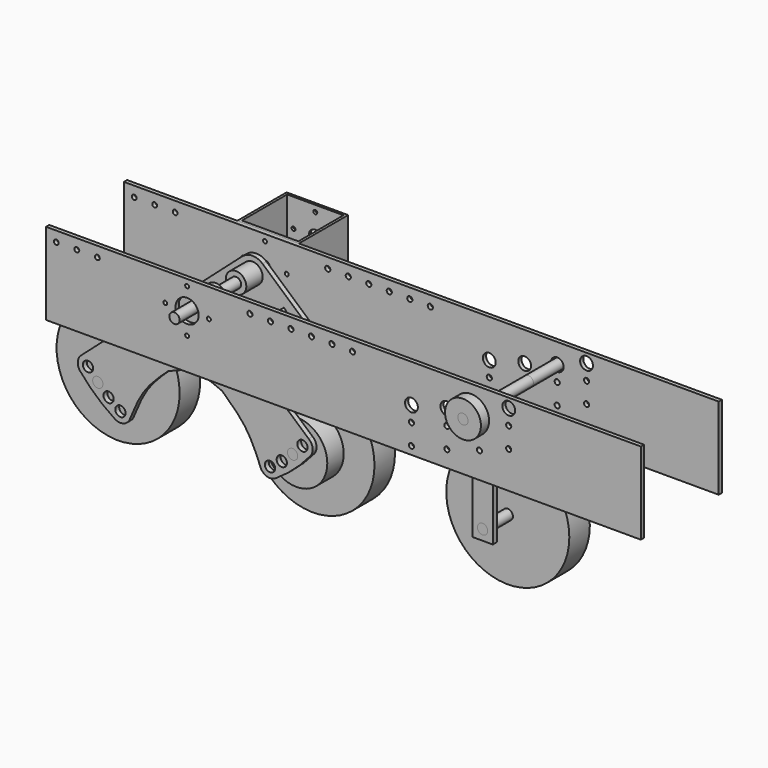
from build123d import *

# Parameters (mm, degrees)
F1_R           = 76.2
F1_R_2         = 6.35
F2_DEPTH       = 31.75
F3_R           = 38.1
F3_R_2         = 6.35
F4_DEPTH       = 25.4
F5_R           = 38.1
F5_R_2         = 6.35
F6_DEPTH       = 25.4
F0_R           = 6.35
F7_DEPTH       = 25.4
F7_DEPTH_BACK  = 57.15
F8_R           = 12.7
F8_R_2         = 6.35
F9_DEPTH       = 25.4
F10_R          = 12.7
F10_R_2        = 6.35
F11_DEPTH      = 25.4
F12_R          = 6.35
F13_DEPTH      = 6.0452
F14_R          = 6.35
F14_R_2        = 3.175
F15_DEPTH      = 6.0452
F18_W          = 736.6
F18_H          = 101.6
F18_R          = 2.4257
F18_R_2        = 3.175
F18_R_3        = 6.35
F18_R_4        = 2.983685919
F18_R_5        = 7.9375
F19_DEPTH      = 4.9403
F21_W          = 736.6
F21_H          = 101.6
F21_R          = 2.4257
F21_R_2        = 3.175
F21_R_3        = 14.2875
F21_R_4        = 2.983685919
F21_R_5        = 7.9375
F22_DEPTH      = 4.9403
F23_R          = 22.225
F24_DEPTH      = 11.43
F26_W          = 25.4
F26_H          = 6.35
F27_DEPTH      = 12.7
F27_DEPTH_BACK = 152.4
F28_R          = 6.35
F28_R_2        = 7.9375
F28_R_3        = 3.175
F29_DEPTH      = 126.8603
F30_W          = 76.2
F30_H          = 76.2
F30_W_2        = 69.85
F30_H_2        = 69.85
F31_DEPTH      = 69.85
F32_R          = 2.4257
F32_R_2        = 7.9375
F33_DEPTH      = 76.2
F34_R          = 6.35
F35_DEPTH      = 56.0451
F35_DEPTH_BACK = 75.7555
F36_DEPTH      = 25.4
F37_R          = 22.225
F37_R_2        = 6.35
F38_DEPTH      = 12.7
F39_DEPTH      = 38.1
F40_R          = 6.35
F41_DEPTH      = 126.8603
F42_R          = 6.35
F43_DEPTH      = 94.6404
F44_DEPTH      = 50.8
F45_R          = 3.175
F46_DEPTH      = 82.55


with BuildPart() as f2:
    # F1 (on Front) → F2 (new body)
    with BuildSketch(Plane.XZ):
        Circle(F1_R)
        Circle(F1_R_2, mode=Mode.SUBTRACT)
    extrude(amount=F2_DEPTH)


with BuildPart() as f2b:
    # F1 (on Front) → F2, piece 2 (new body)
    with BuildSketch(Plane.XZ):
        with Locations((241.3, 0)):
            Circle(F1_R)
        with Locations((241.3, 0)):
            Circle(F1_R_2, mode=Mode.SUBTRACT)
    extrude(amount=F2_DEPTH)


with BuildPart() as f2c:
    # F1 (on Front) → F2, piece 3 (new body)
    with BuildSketch(Plane.XZ):
        with Locations((482.6, 0.0227596388)):
            Circle(F1_R)
        with Locations((482.6, 0.0227596388)):
            Circle(F1_R_2, mode=Mode.SUBTRACT)
    extrude(amount=F2_DEPTH)


with BuildPart() as f4:
    # F3 (on face) → F4 (new body)
    with BuildSketch(Plane.XZ):
        Circle(F3_R)
        Circle(F3_R_2, mode=Mode.SUBTRACT)
    extrude(amount=-F4_DEPTH)


with BuildPart() as f6:
    # F5 (on face) → F6 (new body)
    with BuildSketch(Plane.XZ.offset(31.75)):
        with Locations((241.3, 0)):
            Circle(F5_R)
        with Locations((241.3, 0)):
            Circle(F5_R_2, mode=Mode.SUBTRACT)
    extrude(amount=F6_DEPTH)


with BuildPart() as f7:
    # F0 (on Front) → F7 (new body, two sides)
    with BuildSketch(Plane.XZ) as f7_sk:
        with Locations((120.65, 122.1713596388)):
            Circle(F0_R)
    extrude(amount=-F7_DEPTH)
    extrude(f7_sk.sketch, amount=F7_DEPTH_BACK)

    # F39 (add): a face of the model
    f39_faces = [f7.faces().sort_by_distance(p)[0] for p in [
        (120.65, -57.15, 122.1713596388),
    ]]
    extrude(f39_faces, amount=F39_DEPTH)


with BuildPart() as f9:
    # F8 (on face) → F9 (new body)
    with BuildSketch(Plane.XZ.offset(57.15)):
        with Locations((120.65, 122.1713596388)):
            Circle(F8_R)
        with Locations((120.65, 122.1713596388)):
            Circle(F8_R_2, mode=Mode.SUBTRACT)
    extrude(amount=-F9_DEPTH)


with BuildPart() as f11:
    # F10 (on face) → F11 (new body)
    with BuildSketch(Plane(origin=(0, 25.4, 0), x_dir=(-1, 0, 0), z_dir=(0, 1, 0))):
        with Locations((-120.65, 122.1713596388)):
            Circle(F10_R)
        with Locations((-120.65, 122.1713596388)):
            Circle(F10_R_2, mode=Mode.SUBTRACT)
    extrude(amount=-F11_DEPTH)


with BuildPart() as f13:
    # F12 (on face) → F13 (new body)
    with BuildSketch(Plane(origin=(0, 25.4, 0), x_dir=(-1, 0, 0), z_dir=(0, 1, 0))):
        with BuildLine():
            Line((-133.2704333117, 136.4411586221), (-261.0948431927, 23.3912521446))
            ThreePointArc((-261.0948431927, 23.3912521446), (-266.0226994754, 14.7625060658), (-263.2289371867, 5.2265782815))
            ThreePointArc((-263.2289371867, 5.2265782815), (-243.1793595629, -15.6378971661), (-220.112702455, -33.1090513484))
            ThreePointArc((-220.112702455, -33.1090513484), (-210.3154284268, -34.7681016947), (-202.3223963934, -28.864673424))
            add(Edge.make_bspline(
                [(-202.3223963934, -28.864673424), (-196.8876219657, -15.4698153256), (-186.0180731103, 11.3199008713), (-164.7164012291, 30.8666336238), (-154.0655652885, 40.64)],
                knots=[0, 0, 0, 0, 0.5, 1, 1, 1, 1], degree=3))
            add(Edge.make_bspline(
                [(-154.0655652885, 40.64), (-142.9270435257, 45.4025), (-120.65, 54.9275), (-98.3729564743, 45.4025), (-87.2344347115, 40.64)],
                knots=[0, 0, 0, 0, 0.5, 1, 1, 1, 1], degree=3))
            add(Edge.make_bspline(
                [(-87.2344347115, 40.64), (-76.5835987709, 30.8666336238), (-55.2819268897, 11.3199008713), (-44.4123780343, -15.4698153256), (-38.9776036066, -28.864673424)],
                knots=[0, 0, 0, 0, 0.5, 1, 1, 1, 1], degree=3))
            ThreePointArc((-38.9776036066, -28.864673424), (-30.9845715732, -34.7681016947), (-21.187297545, -33.1090513484))
            ThreePointArc((-21.187297545, -33.1090513484), (1.8793595629, -15.6378971661), (21.9289371867, 5.2265782815))
            ThreePointArc((21.9289371867, 5.2265782815), (24.7226994754, 14.7625060658), (19.7948431927, 23.3912521446))
            Line((19.7948431927, 23.3912521446), (-108.0295666883, 136.4411586221))
            ThreePointArc((-108.0295666883, 136.4411586221), (-120.65, 141.2213596388), (-133.2704333117, 136.4411586221))
        make_face()
        with Locations((-213.2626540765, -22.4148081674)):
            Circle(F12_R, mode=Mode.SUBTRACT)
        with Locations((-241.3, 0)):
            Circle(F12_R, mode=Mode.SUBTRACT)
        with Locations((-227.8686821978, -11.9420916021)):
            Circle(F12_R, mode=Mode.SUBTRACT)
        with Locations((-253.4094511545, 13.2806265843)):
            Circle(F12_R, mode=Mode.SUBTRACT)
        with Locations((-28.0373459235, -22.4148081674)):
            Circle(F12_R, mode=Mode.SUBTRACT)
        with Locations((-13.4313178022, -11.9420916021)):
            Circle(F12_R, mode=Mode.SUBTRACT)
        Circle(F12_R, mode=Mode.SUBTRACT)
        with Locations((12.1094511545, 13.2806265843)):
            Circle(F12_R, mode=Mode.SUBTRACT)
        with Locations((-120.65, 122.1713596388)):
            Circle(F12_R, mode=Mode.SUBTRACT)
    extrude(amount=F13_DEPTH)


with BuildPart() as f15:
    # F14 (on face) → F15 (new body)
    with BuildSketch(Plane.XZ.offset(57.15)):
        with BuildLine():
            ThreePointArc((133.2704333117, 136.4411586221), (120.65, 141.2213596388), (108.0295666883, 136.4411586221))
            Line((108.0295666883, 136.4411586221), (-19.7948431927, 23.3912521446))
            ThreePointArc((-19.7948431927, 23.3912521446), (-24.7226994754, 14.7625060658), (-21.9289371867, 5.2265782815))
            ThreePointArc((-21.9289371867, 5.2265782815), (-1.8793595629, -15.6378971661), (21.187297545, -33.1090513484))
            ThreePointArc((21.187297545, -33.1090513484), (30.9845715732, -34.7681016947), (38.9776036066, -28.864673424))
            add(Edge.make_bspline(
                [(38.9776036066, -28.864673424), (44.4123780343, -15.4698153256), (55.2819268897, 11.3199008713), (76.5835987709, 30.8666336238), (87.2344347115, 40.64)],
                knots=[0, 0, 0, 0, 0.5, 1, 1, 1, 1], degree=3))
            add(Edge.make_bspline(
                [(87.2344347115, 40.64), (98.3729564743, 45.4025), (120.65, 54.9275), (142.9270435257, 45.4025), (154.0655652885, 40.64)],
                knots=[0, 0, 0, 0, 0.5, 1, 1, 1, 1], degree=3))
            add(Edge.make_bspline(
                [(154.0655652885, 40.64), (164.7164012291, 30.8666336238), (186.0180731103, 11.3199008713), (196.8876219657, -15.4698153256), (202.3223963934, -28.864673424)],
                knots=[0, 0, 0, 0, 0.5, 1, 1, 1, 1], degree=3))
            ThreePointArc((202.3223963934, -28.864673424), (210.3154284268, -34.7681016947), (220.112702455, -33.1090513484))
            ThreePointArc((220.112702455, -33.1090513484), (243.1793595629, -15.6378971661), (263.2289371867, 5.2265782815))
            ThreePointArc((263.2289371867, 5.2265782815), (266.0226994754, 14.7625060658), (261.0948431927, 23.3912521446))
            Line((261.0948431927, 23.3912521446), (133.2704333117, 136.4411586221))
        make_face()
        with Locations((28.0373459235, -22.4148081674)):
            Circle(F14_R, mode=Mode.SUBTRACT)
        Circle(F14_R, mode=Mode.SUBTRACT)
        with Locations((13.4313178022, -11.9420916021)):
            Circle(F14_R, mode=Mode.SUBTRACT)
        with Locations((-12.1094511545, 13.2806265843)):
            Circle(F14_R, mode=Mode.SUBTRACT)
        with Locations((213.2626540765, -22.4148081674)):
            Circle(F14_R, mode=Mode.SUBTRACT)
        with Locations((227.8686821978, -11.9420916021)):
            Circle(F14_R, mode=Mode.SUBTRACT)
        with Locations((241.3, 0)):
            Circle(F14_R, mode=Mode.SUBTRACT)
        with Locations((253.4094511545, 13.2806265843)):
            Circle(F14_R, mode=Mode.SUBTRACT)
        with Locations((65.7991565264, 60.479484402)):
            Circle(F14_R_2, mode=Mode.SUBTRACT)
        with Locations((82.6763391337, 79.4615998595)):
            Circle(F14_R_2, mode=Mode.SUBTRACT)
        with Locations((99.5535217409, 98.443715317)):
            Circle(F14_R_2, mode=Mode.SUBTRACT)
        with Locations((120.65, 122.1713596388)):
            Circle(F14_R, mode=Mode.SUBTRACT)
        with Locations((175.5008434736, 60.479484402)):
            Circle(F14_R_2, mode=Mode.SUBTRACT)
        with Locations((158.6236608663, 79.4615998595)):
            Circle(F14_R_2, mode=Mode.SUBTRACT)
        with Locations((141.7464782591, 98.443715317)):
            Circle(F14_R_2, mode=Mode.SUBTRACT)
    extrude(amount=F15_DEPTH)


with BuildPart() as f19:
    # F18 (on offset) → F19 (new body)
    with BuildSketch(Plane.XZ.offset(-44.7548)):
        with Locations((314.325, 106.2963596388)):
            Rectangle(F18_W, F18_H)
        with Locations((120.65, 95.1838596388)):
            Circle(F18_R, mode=Mode.SUBTRACT)
        with Locations((398.4861859235, 65.4437918326)):
            Circle(F18_R_2, mode=Mode.SUBTRACT)
        with Locations((442.3052378022, 75.9165083979)):
            Circle(F18_R_2, mode=Mode.SUBTRACT)
        with Locations((398.4861859235, 90.8437918326)):
            Circle(F18_R_2, mode=Mode.SUBTRACT)
        with Locations((482.6, 87.8586)):
            Circle(F18_R_2, mode=Mode.SUBTRACT)
        with Locations((442.3052378022, 101.3165083979)):
            Circle(F18_R_2, mode=Mode.SUBTRACT)
        with Locations((518.9283488455, 101.1392265843)):
            Circle(F18_R_2, mode=Mode.SUBTRACT)
        with Locations((93.6625, 122.1713596388)):
            Circle(F18_R, mode=Mode.SUBTRACT)
        with Locations((120.65, 122.1713596388)):
            Circle(F18_R_3, mode=Mode.SUBTRACT)
        with Locations((147.6375, 122.1713596388)):
            Circle(F18_R, mode=Mode.SUBTRACT)
        with Locations((-41.275, 144.3963596388)):
            Circle(F18_R_4, mode=Mode.SUBTRACT)
        with Locations((-15.875, 144.3963596388)):
            Circle(F18_R_4, mode=Mode.SUBTRACT)
        with Locations((9.525, 144.3963596388)):
            Circle(F18_R_4, mode=Mode.SUBTRACT)
        with Locations((120.65, 149.1588596388)):
            Circle(F18_R, mode=Mode.SUBTRACT)
        with Locations((198.4375, 144.3963596388)):
            Circle(F18_R_2, mode=Mode.SUBTRACT)
        with Locations((223.8375, 144.3963596388)):
            Circle(F18_R_2, mode=Mode.SUBTRACT)
        with Locations((249.2375, 144.3963596388)):
            Circle(F18_R_2, mode=Mode.SUBTRACT)
        with Locations((274.6375, 144.3963596388)):
            Circle(F18_R_2, mode=Mode.SUBTRACT)
        with Locations((300.0375, 144.3963596388)):
            Circle(F18_R_2, mode=Mode.SUBTRACT)
        with Locations((398.4861859235, 109.8937918326)):
            Circle(F18_R_5, mode=Mode.SUBTRACT)
        with Locations((482.6, 113.2586)):
            Circle(F18_R_2, mode=Mode.SUBTRACT)
        with Locations((442.3052378022, 120.3665083979)):
            Circle(F18_R_5, mode=Mode.SUBTRACT)
        with Locations((518.9283488455, 126.5392265843)):
            Circle(F18_R_2, mode=Mode.SUBTRACT)
        with Locations((482.6, 132.3086)):
            Circle(F18_R_5, mode=Mode.SUBTRACT)
        with Locations((325.4375, 144.3963596388)):
            Circle(F18_R_2, mode=Mode.SUBTRACT)
        with Locations((518.9283488455, 145.5892265843)):
            Circle(F18_R_5, mode=Mode.SUBTRACT)
    extrude(amount=-F19_DEPTH)


with BuildPart() as f22:
    # F21 (on offset) → F22 (new body)
    with BuildSketch(Plane.XZ.offset(70.8152)):
        with Locations((314.325, 106.2963596388)):
            Rectangle(F21_W, F21_H)
        with Locations((120.65, 95.1838596388)):
            Circle(F21_R, mode=Mode.SUBTRACT)
        with Locations((398.4861859235, 65.4437918326)):
            Circle(F21_R_2, mode=Mode.SUBTRACT)
        with Locations((442.3052378022, 75.9165083979)):
            Circle(F21_R_2, mode=Mode.SUBTRACT)
        with Locations((398.4861859235, 90.8437918326)):
            Circle(F21_R_2, mode=Mode.SUBTRACT)
        with Locations((482.6, 87.8586)):
            Circle(F21_R_2, mode=Mode.SUBTRACT)
        with Locations((442.3052378022, 101.3165083979)):
            Circle(F21_R_2, mode=Mode.SUBTRACT)
        with Locations((518.9283488455, 101.1392265843)):
            Circle(F21_R_2, mode=Mode.SUBTRACT)
        with Locations((93.6625, 122.1713596388)):
            Circle(F21_R, mode=Mode.SUBTRACT)
        with Locations((120.65, 122.1713596388)):
            Circle(F21_R_3, mode=Mode.SUBTRACT)
        with Locations((147.6375, 122.1713596388)):
            Circle(F21_R, mode=Mode.SUBTRACT)
        with Locations((-41.275, 144.3963596388)):
            Circle(F21_R_4, mode=Mode.SUBTRACT)
        with Locations((-15.875, 144.3963596388)):
            Circle(F21_R_4, mode=Mode.SUBTRACT)
        with Locations((9.525, 144.3963596388)):
            Circle(F21_R_4, mode=Mode.SUBTRACT)
        with Locations((120.65, 149.1588596388)):
            Circle(F21_R, mode=Mode.SUBTRACT)
        with Locations((198.4375, 144.3963596388)):
            Circle(F21_R_2, mode=Mode.SUBTRACT)
        with Locations((223.8375, 144.3963596388)):
            Circle(F21_R_2, mode=Mode.SUBTRACT)
        with Locations((249.2375, 144.3963596388)):
            Circle(F21_R_2, mode=Mode.SUBTRACT)
        with Locations((274.6375, 144.3963596388)):
            Circle(F21_R_2, mode=Mode.SUBTRACT)
        with Locations((300.0375, 144.3963596388)):
            Circle(F21_R_2, mode=Mode.SUBTRACT)
        with Locations((398.4861859235, 109.8937918326)):
            Circle(F21_R_5, mode=Mode.SUBTRACT)
        with Locations((482.6, 113.2586)):
            Circle(F21_R_2, mode=Mode.SUBTRACT)
        with Locations((442.3052378022, 120.3665083979)):
            Circle(F21_R_5, mode=Mode.SUBTRACT)
        with Locations((518.9283488455, 126.5392265843)):
            Circle(F21_R_2, mode=Mode.SUBTRACT)
        with Locations((482.6, 132.3086)):
            Circle(F21_R_5, mode=Mode.SUBTRACT)
        with Locations((325.4375, 144.3963596388)):
            Circle(F21_R_2, mode=Mode.SUBTRACT)
        with Locations((518.9283488455, 145.5892265843)):
            Circle(F21_R_5, mode=Mode.SUBTRACT)
    extrude(amount=F22_DEPTH)


with BuildPart() as f24:
    # F23 (on face) → F24 (new body)
    with BuildSketch(Plane.XZ):
        with Locations((482.6, 0.0227596388)):
            Circle(F23_R)
    extrude(amount=-F24_DEPTH)


with BuildPart() as f27:
    # F26 (on plane+point) → F27 (new body, two sides)
    with BuildSketch(Plane(origin=(0, 0, 0.0227596388), x_dir=(1, 0, 0), z_dir=(0, 0, -1))) as f27_sk:
        with Locations((482.6, -52.8701)):
            Rectangle(F26_W, F26_H)
    extrude(amount=F27_DEPTH)
    extrude(f27_sk.sketch, amount=-F27_DEPTH_BACK)


with BuildPart() as f27b:
    # F26 (on plane+point) → F27, piece 2 (new body, two sides)
    with BuildSketch(Plane(origin=(0, 0, 0.0227596388), x_dir=(1, 0, 0), z_dir=(0, 0, -1))) as f27_2_sk:
        with Locations((482.6, 67.6402)):
            Rectangle(F26_W, F26_H)
    extrude(amount=F27_DEPTH)
    extrude(f27_2_sk.sketch, amount=-F27_DEPTH_BACK)


with BuildPart() as f29_tool:
    # F28 (on face) → F29 (new body, through all)
    with BuildSketch(Plane.XZ.offset(70.8152)):
        with Locations((482.6, 0.0227596388)):
            Circle(F28_R)
        with Locations((482.6, 132.3086)):
            Circle(F28_R_2)
        with Locations((482.6, 113.2586)):
            Circle(F28_R_3)
        with Locations((482.6, 87.8586)):
            Circle(F28_R_3)
    extrude(amount=-F29_DEPTH)


with BuildPart() as f24_1:
    add(f24.part)

    # F29: cut by f29_tool
    add(f29_tool.part, mode=Mode.SUBTRACT)


with BuildPart() as f27_1:
    add(f27.part)

    # F29: cut by f29_tool
    add(f29_tool.part, mode=Mode.SUBTRACT)


with BuildPart() as f27b_1:
    add(f27b.part)

    # F29: cut by f29_tool
    add(f29_tool.part, mode=Mode.SUBTRACT)


with BuildPart() as f31:
    # F30 (on face) → F31 (new body)
    with BuildSketch(Plane.XY.offset(157.0963596388)):
        with Locations((120.65, 87.7951)):
            Rectangle(F30_W, F30_H)
        with Locations((120.65, 87.7951)):
            Rectangle(F30_W_2, F30_H_2, mode=Mode.SUBTRACT)
    extrude(amount=-F31_DEPTH)

    # F32 (on face) → F33 (cut, through all)
    with BuildSketch(Plane(origin=(0, 125.8951, 0), x_dir=(-1, 0, 0), z_dir=(0, 1, 0))):
        with Locations((-120.65, 149.1588596388)):
            Circle(F32_R)
        with Locations((-147.6375, 122.1713596388)):
            Circle(F32_R)
        with Locations((-120.65, 95.1838596388)):
            Circle(F32_R)
        with Locations((-93.6625, 122.1713596388)):
            Circle(F32_R)
        with Locations((-120.65, 122.1713596388)):
            Circle(F32_R_2)
    extrude(amount=-F33_DEPTH, mode=Mode.SUBTRACT)


with BuildPart() as f35:
    # F34 (on Front) → F35 (new body, two sides)
    with BuildSketch(Plane.XZ) as f35_sk:
        with Locations((482.6, 132.3086)):
            Circle(F34_R)
    extrude(amount=-F35_DEPTH)
    extrude(f35_sk.sketch, amount=F35_DEPTH_BACK)

    # F36 (add): a face of the model
    f36_faces = [f35.faces().sort_by_distance(p)[0] for p in [
        (482.6, -75.7555, 132.3086),
    ]]
    extrude(f36_faces, amount=F36_DEPTH)


with BuildPart() as f38:
    # F37 (on face) → F38 (new body)
    with BuildSketch(Plane.XZ.offset(101.1555)):
        with Locations((482.6, 132.3086)):
            Circle(F37_R)
        with Locations((482.6, 132.3086)):
            Circle(F37_R_2, mode=Mode.SUBTRACT)
    extrude(amount=-F38_DEPTH)


with BuildPart() as f41:
    # F40 (on face) → F41 (new body, through all)
    with BuildSketch(Plane.XZ.offset(70.8152)):
        with Locations((482.6, 0.0227596388)):
            Circle(F40_R)
    extrude(amount=-F41_DEPTH)


with BuildPart() as f43:
    # F42 (on face) → F43 (new body, through all)
    with BuildSketch(Plane.XZ.offset(63.1952)):
        Circle(F42_R)
    extrude(amount=-F43_DEPTH)


with BuildPart() as f43b:
    # F42 (on face) → F43, piece 2 (new body, through all)
    with BuildSketch(Plane.XZ.offset(63.1952)):
        with Locations((241.3, 0)):
            Circle(F42_R)
    extrude(amount=-F43_DEPTH)


with BuildPart() as f44:
    # F44 (new): a face of the model
    f44_faces = [f7.part.faces().sort_by_distance(p)[0] for p in [
        (120.65, 25.4, 122.1713596388),
    ]]
    extrude(f44_faces, amount=F44_DEPTH)


with BuildPart() as f46:
    # F45 (on face) → F46 (new body, through all)
    with BuildSketch(Plane(origin=(0, -57.15, 0), x_dir=(-1, 0, 0), z_dir=(0, 1, 0))):
        Polygon((-159.6761272914, 97.3912488918), (-193.4304925059, 59.4270179769), (-174.4483770484, 42.5498353696), (-140.6940118339, 80.5140662846), align=None)
        with Locations((-175.5008434736, 60.479484402)):
            Circle(F45_R, mode=Mode.SUBTRACT)
        with Locations((-158.6236608663, 79.4615998595)):
            Circle(F45_R, mode=Mode.SUBTRACT)
    extrude(amount=F46_DEPTH)


solid = Compound([f2.part, f2b.part, f2c.part, f4.part, f6.part, f7.part, f9.part, f11.part, f13.part, f15.part, f19.part, f22.part, f24_1.part, f27_1.part, f27b_1.part, f31.part, f35.part, f38.part, f41.part, f43.part, f43b.part, f44.part, f46.part])
